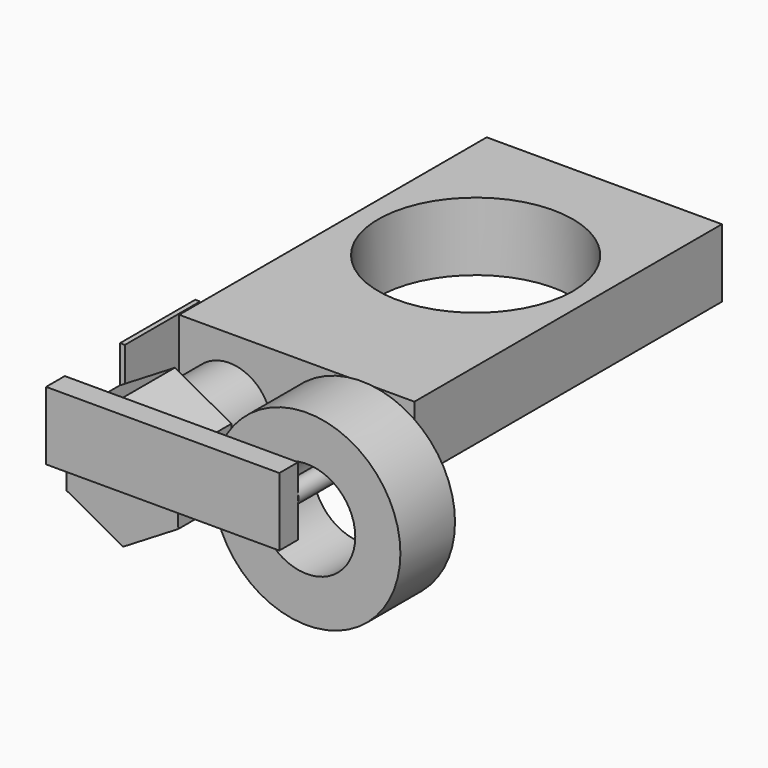
from build123d import *

# Parameters (mm, degrees)
F1_DEPTH     = 25.4
F2_R         = 25.8999671589
F2_R_2       = 17.2023355416
F3_DEPTH     = 25.4
F4_R         = 34.8318560705
F4_R_2       = 18.0308272553
F5_DEPTH     = 25.4
F6_R         = 14.9551436637
F7_DEPTH     = 25.4
F8_R         = 15.7218012702
F9_DEPTH     = 25.4
F10_W        = 87.5383242965
F10_H        = 13.5084241629
F11_DEPTH    = 25.4
F12_R        = 3.589274675
F13_DEPTH    = 25.4
F15_DEPTH    = 129.54
F16_DEPTH    = 25.4
F17_W        = 86.8061985821
F17_H        = 8.7011847645
F18_DEPTH    = 25.4
F19_R        = 36.2307294495
F20_DEPTH    = 25.4
F21_T        = 2.54
F21_T6_ANGLE = 180.000000001
F22_W        = 1.8093809485
F22_H        = 34.9651761353
F23_DEPTH    = 25.4


# Not quite as in the source:
# - a shell that OpenCascade refuses in one call is made with other operations: the cavity is built on its own and cut out


with BuildPart() as f1:
    # F0 (on Front) → F1 (new body)
    with BuildSketch(Plane.XZ):
        Polygon((-48.3754668356, 12.4674958523), (-69.4210231304, 23.9844769239), (-89.9177994608, 11.5169810717), (-89.3690194964, -12.4674958523), (-68.3234632015, -23.9844769239), (-47.8266868711, -11.5169810717), align=None)
    extrude(amount=F1_DEPTH)

    # F2 (on Front) → F3 (cut)
    with BuildSketch(Plane.XZ):
        Circle(F2_R)
        Circle(F2_R_2, mode=Mode.SUBTRACT)
        Circle(F2_R_2)
    extrude(amount=-F3_DEPTH, mode=Mode.SUBTRACT)

    # F6 (on Front) → F7 (join)
    with BuildSketch(Plane.XZ):
        with Locations((-68.4596300125, 0)):
            Circle(F6_R)
    extrude(amount=F7_DEPTH)

    # F8 (on face) → F9 (join)
    with BuildSketch(Plane(origin=(0, 0, 0), x_dir=(-1, 0, 0), z_dir=(0, 1, 0))):
        with Locations((68.9029097557, 0)):
            Circle(F8_R)
    extrude(amount=F9_DEPTH)

    # F10 (on Top) → F11 (join)
    with BuildSketch(Plane.XY):
        with Locations((-43.7691621482, 31.4080566168)):
            Rectangle(F10_W, F10_H)
    extrude(amount=F11_DEPTH)

    # F12 (on face) → F13 (join)
    with BuildSketch(Plane.XZ.offset(-24.6538445354)):
        with Locations((-6.0427188873, 13.5841108859)):
            Circle(F12_R)
    extrude(amount=F13_DEPTH)

    # F14 (on face) → F15 (join)
    with BuildSketch(Plane(origin=(0, 38.1622686982, 0), x_dir=(-1, 0, 0), z_dir=(0, 1, 0))):
        Polygon((49.9359071255, 0), (87.5383242965, 0), (87.5383242965, 25.4), (0, 25.4), (0, 0), align=None)
    extrude(amount=F15_DEPTH)

    # F16 (add): a face of the model
    f16_faces = [f1.faces().sort_by_distance(p)[0] for p in [
        (-6.0427188873, -0.7461554646, 13.5841108859),
    ]]
    extrude(f16_faces, amount=F16_DEPTH)

    # F19 (on face) → F20 (cut)
    with BuildSketch(Plane.XY.offset(25.4)):
        with Locations((-43.7086820602, 107.7667698264)):
            Circle(F19_R)
    extrude(amount=-F20_DEPTH, mode=Mode.SUBTRACT)

    # F21: shell of thickness 2.54, made by hand


with BuildPart() as f5:
    # F4 (on Front) → F5 (new body)
    with BuildSketch(Plane.XZ):
        with Locations((0, 7.3354803026)):
            Circle(F4_R)
        with Locations((0, 7.3354803026)):
            Circle(F4_R_2, mode=Mode.SUBTRACT)
    extrude(amount=F5_DEPTH)


with BuildPart() as f18:
    # F17 (on Top) → F18 (new body)
    with BuildSketch(Plane.XY):
        with Locations((-46.0046427324, -30.5737545714)):
            Rectangle(F17_W, F17_H)
    extrude(amount=F18_DEPTH)


with BuildPart() as f21_core1:
    # F21_t2: copy of F1
    add(f1.part)

    # the walls: a layer under each face that stays
    f21_faces = [f21_core1.faces().sort_by_distance(p)[0] for p in [
        (-58.898244983, -12.7, 18.2259863881),
        (-48.1010768534, -12.7, 0.4752573903),
        (-79.6694112956, -12.7, 17.7507289978),
        (-82.9026140292, 0, -15.9896512826),
        (-68.872243166, -25.4, 0),
        (-58.0750750363, -12.7, -17.7507289978),
        (-89.6434094786, -12.7, -0.4752573903),
        (-78.8462413489, -12.7, -18.2259863881),
        (-53.1811084855, 12.7, 0),
        (-68.9029097557, 25.4, -7.8609006351),
        (-43.7691621482, 24.6538445354, 12.7),
        (0, 96.1780566168, 12.7),
        (-43.7691621482, 167.7022686982, 12.7),
        (-87.5383242965, 96.1780566168, 12.7),
        (-79.9394115097, 107.7667698264, 12.7),
        (-72.9486035804, 48.4952485625, 25.4),
        (-9.6319935623, -0.7461554646, 13.5841108859),
        (-6.0427188873, -26.1461554646, 13.5841108859),
    ]]
    thicken(f21_faces, amount=-F21_T, mode=Mode.SUBTRACT)

    # F21_s3 → F21_t4 (revolve, cut)
    with BuildSketch(Plane.XY):
        Polygon((-84.6501110259, 0.0254), (-84.6247110259, -2.54), (-82.0847110259, -2.54), (-82.0847110259, 0), align=None)
    revolve(axis=Axis((-68.9029097557, 0, 0), (0, 1, 0)), mode=Mode.SUBTRACT)

    # F21_s5 → F21_t6 (revolve, cut)
    with BuildSketch(Plane.XY):
        Polygon((-53.1557084855, 24.6284445354), (-55.7211084855, 24.6538445354), (-55.7211084855, 27.1938445354), (-53.1811084855, 27.1938445354), align=None)
    revolve(axis=Axis((-68.9029097557, 24.6538445354, 0), (0, -1, 0)), revolution_arc=F21_T6_ANGLE, mode=Mode.SUBTRACT)

    # F21_s7 → F21_t8 (revolve, cut)
    with BuildSketch(Plane.XY.offset(13.5841108859)):
        Polygon((-2.4280442124, 24.6284445354), (-2.4534442124, 27.1938445354), (-4.9934442124, 27.1938445354), (-4.9934442124, 24.6538445354), align=None)
    revolve(axis=Axis((-6.0427188873, 24.6538445354, 13.5841108859), (0, -1, 0)), mode=Mode.SUBTRACT)


with BuildPart() as f1_1:
    add(f1.part)

    # what is left inside the walls is the cavity
    f21_cavity = [f21_core1.part.solids().sort_by_distance(p)[0] for p in [
        (-64.383743, 38.671363, 0.0254),
    ]]
    add(f21_cavity, mode=Mode.SUBTRACT)

    # F22 (on Top) → F23 (join)
    with BuildSketch(Plane.XY):
        with Locations((-88.920827955, 17.4825880677)):
            Rectangle(F22_W, F22_H)
    extrude(amount=F23_DEPTH)


solid = Compound([f5.part, f18.part, f1_1.part])
